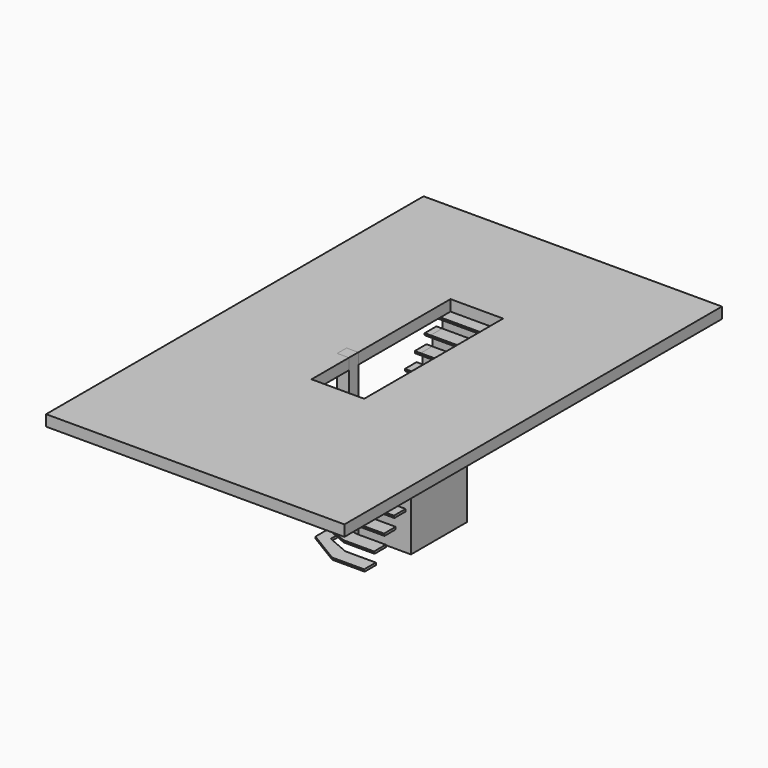
from build123d import *

# Parameters (mm, degrees)
F2_W        = 5100.8088588715
F2_H        = 8066.695690155
F2_W_2      = 900
F2_H_2      = 2970
F3_DEPTH    = 188
F4_W        = 200
F4_H        = 200
F5_DEPTH    = 2750
F9_DEPTH    = 900
F10_DEPTH   = 100
F12_DEPTH   = 900
F13_DEPTH   = 50
F18_DEPTH   = 40
F20_DEPTH   = 40
F22_DEPTH   = 40
F33_SIZE    = 10
F33_2_SIZE  = 10
F33_3_SIZE  = 10
F33_4_SIZE  = 10
F33_5_SIZE  = 10
F33_6_SIZE  = 10
F33_7_SIZE  = 10
F33_8_SIZE  = 10
F33_9_SIZE  = 10
F33_10_SIZE = 10
F33_11_SIZE = 10
F33_12_SIZE = 10
F33_13_SIZE = 10
F33_14_SIZE = 10
F33_15_SIZE = 10
F33_16_SIZE = 10
F33_17_SIZE = 10
F33_18_SIZE = 10
F33_19_SIZE = 10
F33_20_SIZE = 10
F33_21_SIZE = 10
F33_22_SIZE = 10
F33_23_SIZE = 10
F33_24_SIZE = 10


# Not quite as in the source:
# - the program builds the solid bodies; features that only make, move or delete a surface that nothing else refers to are left out


with BuildPart() as f3:
    # F2 (on offset) → F3 (new body)
    with BuildSketch(Plane.XY.offset(2750)):
        with Locations((-487.065911293, 232.9032421112)):
            Rectangle(F2_W, F2_H)
        with Locations((-450, 685)):
            Rectangle(F2_W_2, F2_H_2, mode=Mode.SUBTRACT)
    extrude(amount=-F3_DEPTH)


with BuildPart() as f5:
    # F4 (on Top) → F5 (new body, through all)
    with BuildSketch(Plane.XY):
        with Locations((-1000, 100)):
            Rectangle(F4_W, F4_H)
    extrude(amount=F5_DEPTH)


with BuildPart() as f9:
    # F8 (on plane+point) → F9 (new body, through all)
    with BuildSketch(Plane.YZ.offset(-900)):
        Polygon((2168, 2562), (1956, 2562), (1956, 2522), (2206, 2522), (2206, 2562), align=None)
    extrude(amount=F9_DEPTH)


with BuildPart() as f9b:
    # F8 (on plane+point) → F9, piece 2 (new body, through all)
    with BuildSketch(Plane.YZ.offset(-900)):
        Polygon((1956, 2379), (1744, 2379), (1744, 2339), (1994, 2339), (1994, 2379), align=None)
    extrude(amount=F9_DEPTH)


with BuildPart() as f9c:
    # F8 (on plane+point) → F9, piece 3 (new body, through all)
    with BuildSketch(Plane.YZ.offset(-900)):
        Polygon((1744, 2196), (1532, 2196), (1532, 2156), (1782, 2156), (1782, 2196), align=None)
    extrude(amount=F9_DEPTH)


with BuildPart() as f9d:
    # F8 (on plane+point) → F9, piece 4 (new body, through all)
    with BuildSketch(Plane.YZ.offset(-900)):
        Polygon((1532, 2013), (1320, 2013), (1320, 1973), (1570, 1973), (1570, 2013), align=None)
    extrude(amount=F9_DEPTH)


with BuildPart() as f9e:
    # F8 (on plane+point) → F9, piece 5 (new body, through all)
    with BuildSketch(Plane.YZ.offset(-900)):
        Polygon((1320, 1830), (1108, 1830), (1108, 1790), (1358, 1790), (1358, 1830), align=None)
    extrude(amount=F9_DEPTH)


with BuildPart() as f9f:
    # F8 (on plane+point) → F9, piece 6 (new body, through all)
    with BuildSketch(Plane.YZ.offset(-900)):
        Polygon((1108, 1647), (896, 1647), (896, 1607), (1146, 1607), (1146, 1647), align=None)
    extrude(amount=F9_DEPTH)


with BuildPart() as f9g:
    # F8 (on plane+point) → F9, piece 7 (new body, through all)
    with BuildSketch(Plane.YZ.offset(-900)):
        Polygon((896, 1464), (684, 1464), (684, 1424), (934, 1424), (934, 1464), align=None)
    extrude(amount=F9_DEPTH)


with BuildPart() as f9h:
    # F8 (on plane+point) → F9, piece 8 (new body, through all)
    with BuildSketch(Plane.YZ.offset(-900)):
        Polygon((684, 1281), (472, 1281), (472, 1241), (722, 1241), (722, 1281), align=None)
    extrude(amount=F9_DEPTH)


with BuildPart() as f9i:
    # F8 (on plane+point) → F9, piece 9 (new body, through all)
    with BuildSketch(Plane.YZ.offset(-900)):
        Polygon((472, 1098), (260, 1098), (260, 1058), (510, 1058), (510, 1098), align=None)
    extrude(amount=F9_DEPTH)


with BuildPart() as f9j:
    # F8 (on plane+point) → F9, piece 10 (new body, through all)
    with BuildSketch(Plane.YZ.offset(-900)):
        Polygon((260, 915), (48, 915), (48, 875), (298, 875), (298, 915), align=None)
    extrude(amount=F9_DEPTH)


with BuildPart() as f9k:
    # F8 (on plane+point) → F9, piece 11 (new body, through all)
    with BuildSketch(Plane.YZ.offset(-900)):
        Polygon((48, 732), (-164, 732), (-164, 692), (86, 692), (86, 732), align=None)
    extrude(amount=F9_DEPTH)


with BuildPart() as f10:
    # F10 (new): a face of the model
    f10_faces = [f9.part.faces().sort_by_distance(p)[0] for p in [
        (-900, 2081, 2542),
    ]]
    extrude(f10_faces, amount=F10_DEPTH)

    # F33
    f33_edges = [f10.edges().sort_by_distance(p)[0] for p in [
        (-950, 1956, 2522),
    ]]
    chamfer(f33_edges, length=F33_SIZE)


with BuildPart() as f10b:
    # F10#2 (new): a face of the model
    f10_2_faces = [f9b.part.faces().sort_by_distance(p)[0] for p in [
        (-900, 1869, 2359),
    ]]
    extrude(f10_2_faces, amount=F10_DEPTH)

    # F33#3
    f33_3_edges = [f10b.edges().sort_by_distance(p)[0] for p in [
        (-950, 1744, 2339),
    ]]
    chamfer(f33_3_edges, length=F33_3_SIZE)


with BuildPart() as f10c:
    # F10#3 (new): a face of the model
    f10_3_faces = [f9c.part.faces().sort_by_distance(p)[0] for p in [
        (-900, 1657, 2176),
    ]]
    extrude(f10_3_faces, amount=F10_DEPTH)

    # F33#5
    f33_5_edges = [f10c.edges().sort_by_distance(p)[0] for p in [
        (-950, 1532, 2156),
    ]]
    chamfer(f33_5_edges, length=F33_5_SIZE)


with BuildPart() as f10d:
    # F10#4 (new): a face of the model
    f10_4_faces = [f9d.part.faces().sort_by_distance(p)[0] for p in [
        (-900, 1445, 1993),
    ]]
    extrude(f10_4_faces, amount=F10_DEPTH)

    # F33#7
    f33_7_edges = [f10d.edges().sort_by_distance(p)[0] for p in [
        (-950, 1320, 1973),
    ]]
    chamfer(f33_7_edges, length=F33_7_SIZE)


with BuildPart() as f10e:
    # F10#5 (new): a face of the model
    f10_5_faces = [f9e.part.faces().sort_by_distance(p)[0] for p in [
        (-900, 1233, 1810),
    ]]
    extrude(f10_5_faces, amount=F10_DEPTH)

    # F33#9
    f33_9_edges = [f10e.edges().sort_by_distance(p)[0] for p in [
        (-950, 1108, 1790),
    ]]
    chamfer(f33_9_edges, length=F33_9_SIZE)


with BuildPart() as f10f:
    # F10#6 (new): a face of the model
    f10_6_faces = [f9f.part.faces().sort_by_distance(p)[0] for p in [
        (-900, 1021, 1627),
    ]]
    extrude(f10_6_faces, amount=F10_DEPTH)

    # F33#11
    f33_11_edges = [f10f.edges().sort_by_distance(p)[0] for p in [
        (-950, 896, 1607),
    ]]
    chamfer(f33_11_edges, length=F33_11_SIZE)


with BuildPart() as f10g:
    # F10#7 (new): a face of the model
    f10_7_faces = [f9g.part.faces().sort_by_distance(p)[0] for p in [
        (-900, 809, 1444),
    ]]
    extrude(f10_7_faces, amount=F10_DEPTH)

    # F33#13
    f33_13_edges = [f10g.edges().sort_by_distance(p)[0] for p in [
        (-950, 684, 1424),
    ]]
    chamfer(f33_13_edges, length=F33_13_SIZE)


with BuildPart() as f10h:
    # F10#8 (new): a face of the model
    f10_8_faces = [f9h.part.faces().sort_by_distance(p)[0] for p in [
        (-900, 597, 1261),
    ]]
    extrude(f10_8_faces, amount=F10_DEPTH)

    # F33#15
    f33_15_edges = [f10h.edges().sort_by_distance(p)[0] for p in [
        (-950, 472, 1241),
    ]]
    chamfer(f33_15_edges, length=F33_15_SIZE)


with BuildPart() as f10i:
    # F10#9 (new): a face of the model
    f10_9_faces = [f9i.part.faces().sort_by_distance(p)[0] for p in [
        (-900, 385, 1078),
    ]]
    extrude(f10_9_faces, amount=F10_DEPTH)

    # F33#17
    f33_17_edges = [f10i.edges().sort_by_distance(p)[0] for p in [
        (-950, 260, 1058),
    ]]
    chamfer(f33_17_edges, length=F33_17_SIZE)


with BuildPart() as f10j:
    # F10#10 (new): a face of the model
    f10_10_faces = [f9j.part.faces().sort_by_distance(p)[0] for p in [
        (-900, 173, 895),
    ]]
    extrude(f10_10_faces, amount=F10_DEPTH)


with BuildPart() as f12:
    # F11 (on plane+point) → F12 (new body, through all)
    with BuildSketch(Plane.YZ.offset(-900)):
        Polygon((298, 1058), (298, 915), (298, 875), (200, 875), (200, 0), (1400, 0), (1400, 1643.2547169811), (1146, 1424), (1146, 1607), (934, 1607), (934, 1464), (934, 1424), (722, 1424), (722, 1281), (722, 1241), (510, 1241), (510, 1098), (510, 1058), align=None)
        Polygon((1146, 1424), (1400, 1643.2547169811), (1400, 1973), (1358, 1973), (1358, 1830), (1358, 1790), (1146, 1790), (1146, 1647), (1146, 1607), align=None)
        Polygon((1400, 1973), (1400, 1643.2547169811), (2206, 2339), (2206, 2522), (1994, 2522), (1994, 2379), (1994, 2339), (1782, 2339), (1782, 2196), (1782, 2156), (1570, 2156), (1570, 2013), (1570, 1973), align=None)
    extrude(amount=F12_DEPTH)


with BuildPart() as f13:
    # F13 (new): a face of the model
    f13_faces = [f9k.part.faces().sort_by_distance(p)[0] for p in [
        (-900, -39, 712),
    ]]
    extrude(f13_faces, amount=F13_DEPTH)

    # F33#21
    f33_21_edges = [f13.edges().sort_by_distance(p)[0] for p in [
        (-925, -164, 692),
        (-950, -39, 692),
    ]]
    chamfer(f33_21_edges, length=F33_21_SIZE)


with BuildPart() as f18:
    # F17 (on plane+point) → F18 (new body)
    with BuildSketch(Plane.XY.offset(549)):
        Polygon((-1000, -266), (-500, -376), (0, -376), (0, -126), (-900, -126), (-900, 0), (-1000, 0), (-1000, -126), align=None)
    extrude(amount=-F18_DEPTH)

    # F33#22
    f33_22_edges = [f18.edges().sort_by_distance(p)[0] for p in [
        (-1000, -133, 509),
        (-750, -321, 509),
        (-250, -376, 509),
    ]]
    chamfer(f33_22_edges, length=F33_22_SIZE)


with BuildPart() as f20:
    # F19 (on plane+point) → F20 (new body)
    with BuildSketch(Plane.XY.offset(366)):
        Polygon((-1050, -366), (-525, -588), (0, -588), (0, -338), (-490.9090909091, -338), (-900, -248), (-900, 0), (-1050, 0), (-1050, -226), align=None)
    extrude(amount=-F20_DEPTH)

    # F33#23
    f33_23_edges = [f20.edges().sort_by_distance(p)[0] for p in [
        (-1050, -183, 326),
        (-787.5, -477, 326),
        (-262.5, -588, 326),
    ]]
    chamfer(f33_23_edges, length=F33_23_SIZE)


with BuildPart() as f22:
    # F21 (on plane+point) → F22 (new body)
    with BuildSketch(Plane.XY.offset(183)):
        Polygon((-1100, -466), (-550, -800), (0, -800), (0, -550), (-520.2702702703, -550), (-900, -389.4285714286), (-900, 0), (-1100, 0), (-1100, -326), align=None)
    extrude(amount=-F22_DEPTH)

    # F33#24
    f33_24_edges = [f22.edges().sort_by_distance(p)[0] for p in [
        (-1100, -233, 143),
        (-825, -633, 143),
        (-275, -800, 143),
    ]]
    chamfer(f33_24_edges, length=F33_24_SIZE)


with BuildPart() as f9_1:
    add(f9.part)

    # F33#2
    f33_2_edges = [f9_1.edges().sort_by_distance(p)[0] for p in [
        (-450, 1956, 2522),
    ]]
    chamfer(f33_2_edges, length=F33_2_SIZE)


with BuildPart() as f9b_1:
    add(f9b.part)

    # F33#4
    f33_4_edges = [f9b_1.edges().sort_by_distance(p)[0] for p in [
        (-450, 1744, 2339),
    ]]
    chamfer(f33_4_edges, length=F33_4_SIZE)


with BuildPart() as f9c_1:
    add(f9c.part)

    # F33#6
    f33_6_edges = [f9c_1.edges().sort_by_distance(p)[0] for p in [
        (-450, 1532, 2156),
    ]]
    chamfer(f33_6_edges, length=F33_6_SIZE)


with BuildPart() as f9d_1:
    add(f9d.part)

    # F33#8
    f33_8_edges = [f9d_1.edges().sort_by_distance(p)[0] for p in [
        (-450, 1320, 1973),
    ]]
    chamfer(f33_8_edges, length=F33_8_SIZE)


with BuildPart() as f9e_1:
    add(f9e.part)

    # F33#10
    f33_10_edges = [f9e_1.edges().sort_by_distance(p)[0] for p in [
        (-450, 1108, 1790),
    ]]
    chamfer(f33_10_edges, length=F33_10_SIZE)


with BuildPart() as f9f_1:
    add(f9f.part)

    # F33#12
    f33_12_edges = [f9f_1.edges().sort_by_distance(p)[0] for p in [
        (-450, 896, 1607),
    ]]
    chamfer(f33_12_edges, length=F33_12_SIZE)


with BuildPart() as f9g_1:
    add(f9g.part)

    # F33#14
    f33_14_edges = [f9g_1.edges().sort_by_distance(p)[0] for p in [
        (-450, 684, 1424),
    ]]
    chamfer(f33_14_edges, length=F33_14_SIZE)


with BuildPart() as f9h_1:
    add(f9h.part)

    # F33#16
    f33_16_edges = [f9h_1.edges().sort_by_distance(p)[0] for p in [
        (-450, 472, 1241),
    ]]
    chamfer(f33_16_edges, length=F33_16_SIZE)


with BuildPart() as f9i_1:
    add(f9i.part)

    # F33#18
    f33_18_edges = [f9i_1.edges().sort_by_distance(p)[0] for p in [
        (-450, 260, 1058),
    ]]
    chamfer(f33_18_edges, length=F33_18_SIZE)


with BuildPart() as f9j_1:
    add(f9j.part)

    # F33#19
    f33_19_edges = [f9j_1.edges().sort_by_distance(p)[0] for p in [
        (-450, 48, 875),
    ]]
    chamfer(f33_19_edges, length=F33_19_SIZE)


with BuildPart() as f9k_1:
    add(f9k.part)

    # F33#20
    f33_20_edges = [f9k_1.edges().sort_by_distance(p)[0] for p in [
        (-450, -164, 692),
    ]]
    chamfer(f33_20_edges, length=F33_20_SIZE)


solid = Compound([f3.part, f5.part, f10.part, f10b.part, f10c.part, f10d.part, f10e.part, f10f.part, f10g.part, f10h.part, f10i.part, f10j.part, f12.part, f13.part, f18.part, f20.part, f22.part, f9_1.part, f9b_1.part, f9c_1.part, f9d_1.part, f9e_1.part, f9f_1.part, f9g_1.part, f9h_1.part, f9i_1.part, f9j_1.part, f9k_1.part])
